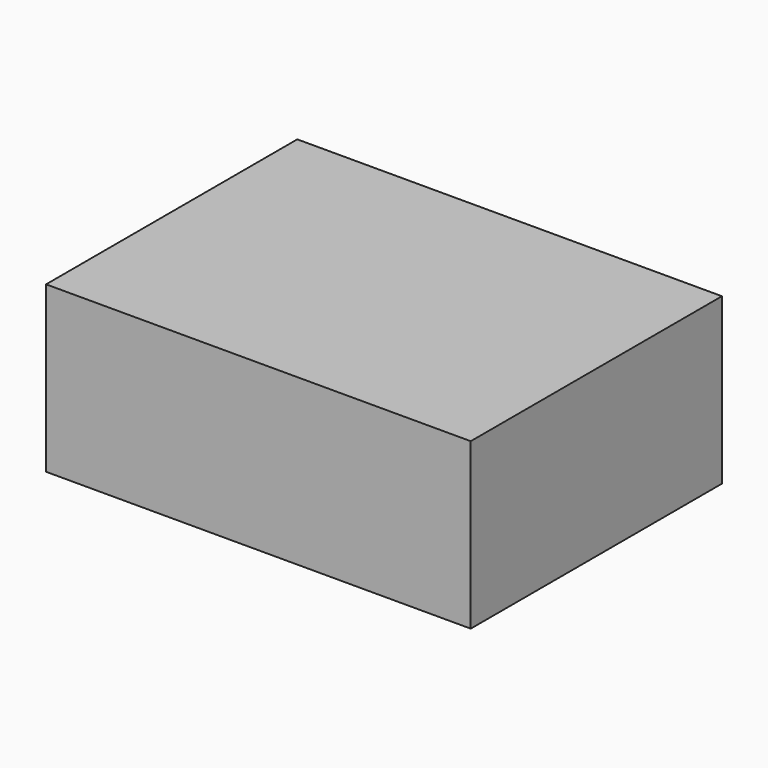
from build123d import *

# Parameters (mm, degrees)
F0_W     = 65.3547011316
F0_H     = 48.3228713274
F1_DEPTH = 25.4


# Not quite as in the source:
# - the program builds the solid bodies; features that only make, move or delete a surface that nothing else refers to are left out


with BuildPart() as f1:
    # F0 (on Top) → F1 (new body)
    with BuildSketch(Plane.XY):
        with Locations((-0.1980457455, -0.5941353738)):
            Rectangle(F0_W, F0_H)
    extrude(amount=F1_DEPTH)


solid = f1.part
